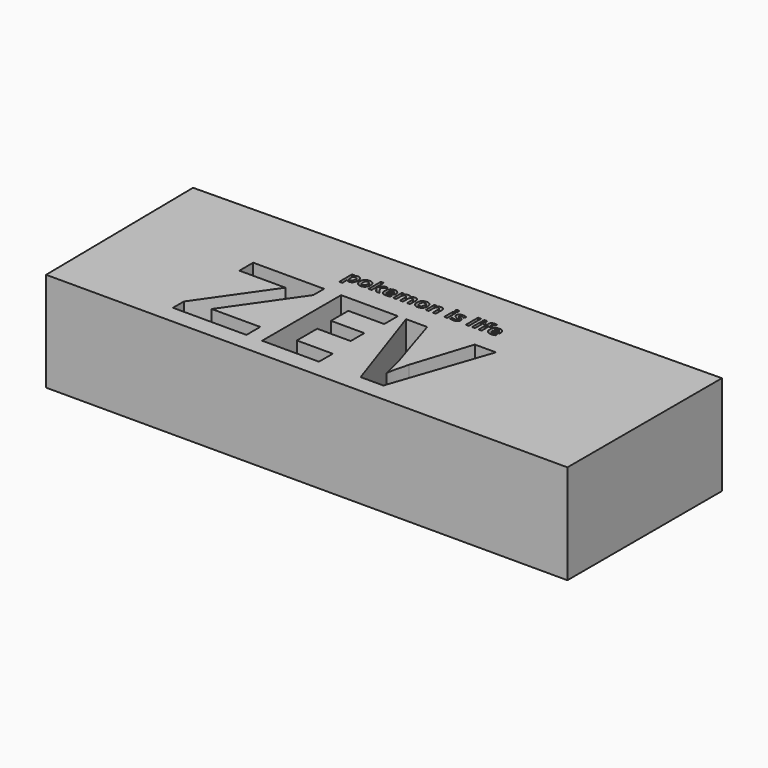
from build123d import *

# Parameters (mm, degrees)
F1_DEPTH     = 25.4
F2_TEXT_SIZE = 35.3292778729
F3_DEPTH     = 25.4
F4_TEXT_SIZE = 5.1856817057
F5_DEPTH     = 25.4


# Not quite as in the source:
# - Text() gives the source's letters only with a copy of the font that has no kerning and outlines rounded to 1/6400 em; it was checked with that copy


with BuildPart() as f1:
    # F0 (on Top) → F1 (new body)
    with BuildSketch(Plane.XY):
        Polygon((68.0701434612, 44.6741483372), (-65.7553999458, 43.0075800868), (-65.1615472924, -4.6788282158), (68.0701434612, -4.6788282158), align=None)
    extrude(amount=F1_DEPTH)

    # F2 (on face) → F3 (cut)
    with BuildSketch(Plane.XY.offset(25.4)):
        with Locations((-37.3260149227, 0)):
            Text('ZEV', F2_TEXT_SIZE, font='Open Sans', font_style=FontStyle.BOLD, text_align=(TextAlign.LEFT, TextAlign.BOTTOM))
    extrude(amount=-F3_DEPTH, mode=Mode.SUBTRACT)

    # F4 (on face) → F5 (cut)
    with BuildSketch(Plane.XY.offset(25.4)):
        with Locations((-18.0044081062, 30.7627916336)):
            Text('pokemon is life', F4_TEXT_SIZE, font='Open Sans', font_style=FontStyle.BOLD, text_align=(TextAlign.LEFT, TextAlign.BOTTOM))
    extrude(amount=-F5_DEPTH, mode=Mode.SUBTRACT)


solid = f1.part
